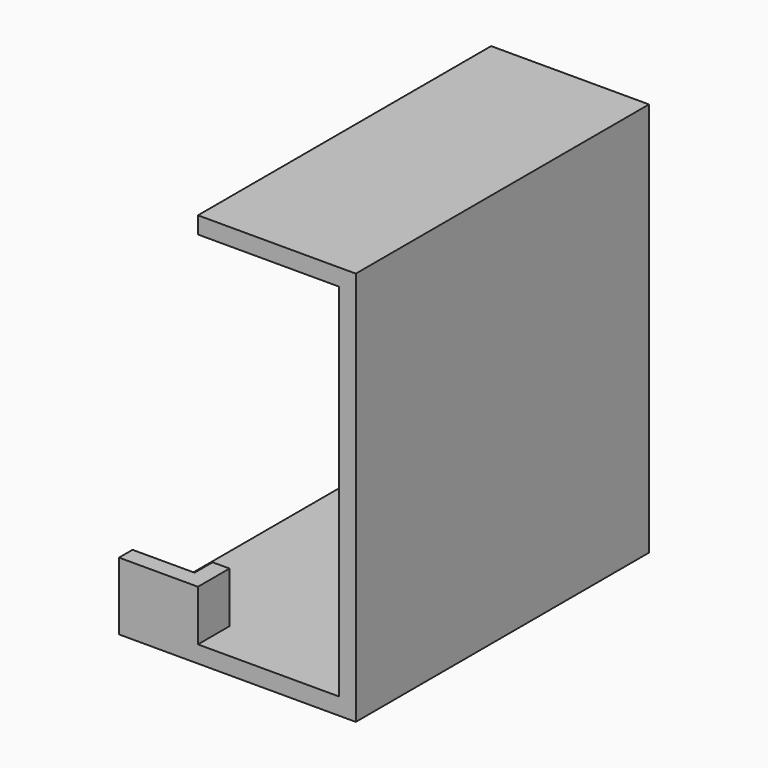
from build123d import *

# Parameters (mm, degrees)
F1_DEPTH = 12
F0_R     = 2
F2_DEPTH = 3
F3_DEPTH = 3
F0_W     = 3
F0_H     = 65
F4_DEPTH = 70
F5_W     = 65
F5_H     = 3
F6_DEPTH = 25


with BuildPart() as f1:
    # F0 (on Top) → F1 (new body)
    with BuildSketch(Plane.XY):
        Polygon((-12.5, 25.5), (-12.5, 32.5), (-26.5, 32.5), (-26.5, 29.5), (-15.5, 29.5), (-15.5, 25.5), align=None)
    extrude(amount=F1_DEPTH)


with BuildPart() as f1b:
    # F0 (on Top) → F1, piece 2 (new body)
    with BuildSketch(Plane.XY):
        Polygon((-12.5, -32.5), (-12.5, -25.5), (-15.5, -25.5), (-15.5, -29.5), (-26.5, -29.5), (-26.5, -32.5), align=None)
    extrude(amount=F1_DEPTH)

    # F0 (on Top) → F2 (join)
    with BuildSketch(Plane.XY):
        Polygon((-12.5, -25.5), (-12.5, 25.5), (-15.5, 25.5), (-15.5, 29.5), (-26.5, 29.5), (-26.5, -29.5), (-15.5, -29.5), (-15.5, -25.5), align=None)
        with Locations((-19.5, -24.5)):
            Circle(F0_R, mode=Mode.SUBTRACT)
        with Locations((-19.5, 24.5)):
            Circle(F0_R, mode=Mode.SUBTRACT)
    extrude(amount=F2_DEPTH)

    # F0 (on Top) → F3 (join)
    with BuildSketch(Plane.XY):
        Polygon((12.5, 32.5), (-12.5, 32.5), (-12.5, 25.5), (-12.5, -25.5), (-12.5, -32.5), (12.5, -32.5), align=None)
    extrude(amount=F3_DEPTH)

    # F0 (on Top) → F4 (join)
    with BuildSketch(Plane.XY):
        with Locations((14, 0)):
            Rectangle(F0_W, F0_H)
    extrude(amount=F4_DEPTH)

    # F5 (on face) → F6 (join)
    with BuildSketch(Plane(origin=(12.5, 0, 0), x_dir=(0, -1, 0), z_dir=(-1, 0, 0))):
        with Locations((0, 68.5)):
            Rectangle(F5_W, F5_H)
    extrude(amount=F6_DEPTH)


solid = Compound([f1.part, f1b.part])
